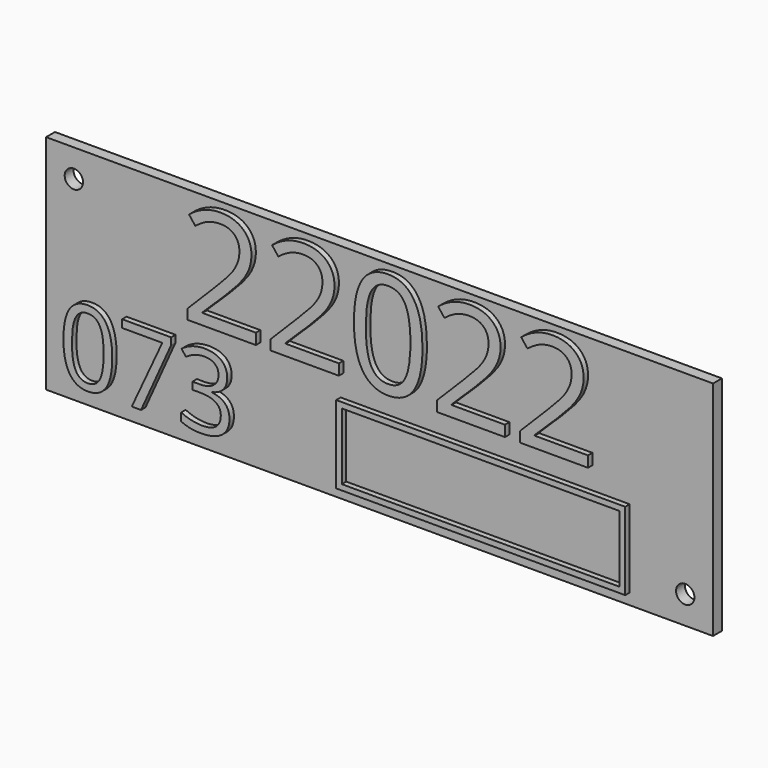
from build123d import *

# Parameters (mm, degrees)
F0_W         = 120
F0_H         = 40
F1_DEPTH     = 2
F3_D         = 3.3
F4_TEXT_SIZE = 26.1338269723
F5_DEPTH     = 1
F6_TEXT_SIZE = 18.5894526641
F7_DEPTH     = 1
F8_W         = 52
F8_H         = 14
F8_W_2       = 49.99999962
F8_H_2       = 11.99999962
F9_DEPTH     = 1


# Not quite as in the source:
# - Text() gives the source's letters only with a copy of the font that has no kerning and outlines rounded to 1/6400 em; it was checked with that copy


with BuildPart() as f1:
    # F0 (on Front) → F1 (new body)
    with BuildSketch(Plane.XZ):
        Rectangle(F0_W, F0_H)
    extrude(amount=F1_DEPTH)

    # F3 (through all)
    with Locations(Plane.XZ.offset(2)):
        with Locations((-55, 15), (55, -15)):
            Hole(F3_D / 2)

    # F4 (on face) → F5 (join)
    with BuildSketch(Plane.XZ.offset(2)):
        with Locations((-35, 0)):
            Text('22022', F4_TEXT_SIZE, font='Open Sans', text_align=(TextAlign.LEFT, TextAlign.BOTTOM))
    extrude(amount=F5_DEPTH)

    # F6 (on face) → F7 (join)
    with BuildSketch(Plane.XZ.offset(2)):
        with Locations((-57, -17)):
            Text('073', F6_TEXT_SIZE, font='Open Sans', text_align=(TextAlign.LEFT, TextAlign.BOTTOM))
    extrude(amount=F7_DEPTH)

    # F8 (on face) → F9 (join)
    with BuildSketch(Plane.XZ.offset(2)):
        with Locations((19, -11)):
            Rectangle(F8_W, F8_H)
        with Locations((19, -11)):
            Rectangle(F8_W_2, F8_H_2, mode=Mode.SUBTRACT)
    extrude(amount=F9_DEPTH)


solid = f1.part
